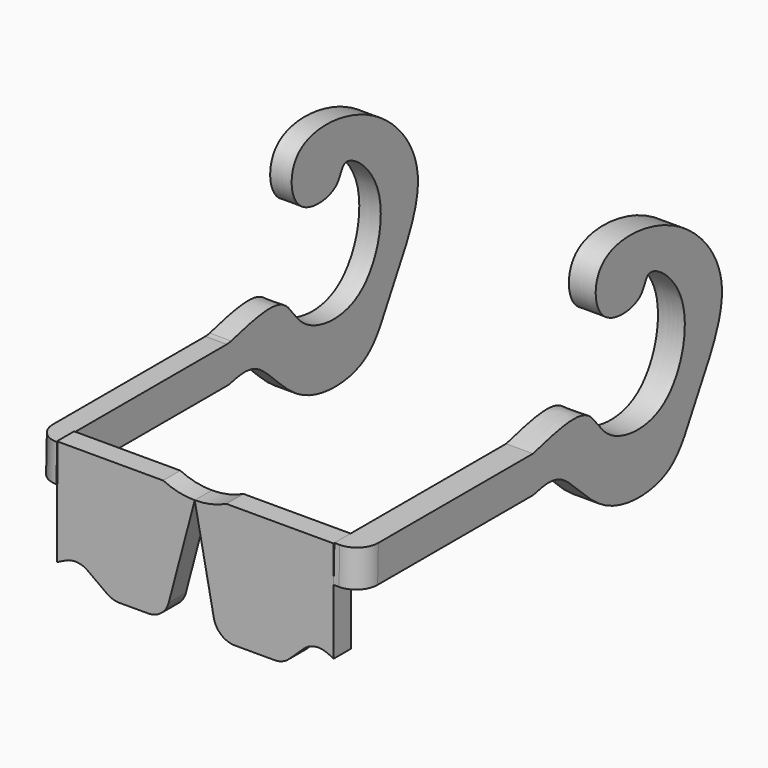
from build123d import *

# Parameters (mm, degrees)
F1_DEPTH  = 5.08
F2_R      = 5.08
F5_DEPTH  = 5.08
F6_R      = 5.08
F7_DEPTH  = 5.08
F8_R      = 5.08
F10_DEPTH = 6.35
F13_R     = 5.07999
F13_2_R   = 5.07999


# Not quite as in the source:
# - a fillet or chamfer is up to 0.001 mm smaller than in the source, because OpenCascade refuses the exact size


with BuildPart() as f1:
    # F0 (on Right) → F1 (new body)
    with BuildSketch(Plane.YZ):
        with BuildLine():
            Line((18.7036339194, 8.6590908468), (-32.0963636041, 8.6590908468))
            Line((-32.0963636041, 8.6590908468), (-32.3272719979, 0))
            Line((-32.3272719979, 0), (18.7036339194, 0))
            add(Edge.make_bspline(
                [(18.7036339194, 0), (21.4167571987, 0.6372428688), (28.063204378, 2.1983223451), (38.2300388432, -13.794123064), (60.394257954, -14.0245683867), (66.1356081474, 0.3511655731), (80.1390378808, 20.7639219103), (62.081530643, 42.703292602), (35.8799194646, 44.0152577696), (37.1192454184, 25.9630287506), (51.7035192179, 26.7390904218), (52.0022911902, 35.2566591152), (67.237499067, 23.591799501), (60.3549528626, -1.2699881146), (39.459302681, 1.5144697653), (35.721169059, 13.1969605328), (24.8370419283, 10.2946159712), (18.7036339194, 8.6590908468)],
                knots=[0, 0, 0, 0, 0.0497967219, 0.1219890317, 0.1968295181, 0.2629995162, 0.3449563898, 0.4313803509, 0.5107878584, 0.5685518225, 0.6256466487, 0.6632894265, 0.7266066585, 0.8065697144, 0.8765027399, 0.9304069977, 1, 1, 1, 1], degree=3))
        make_face()
    extrude(amount=F1_DEPTH)

    # F2
    f2_edges = [f1.edges().sort_by_distance(p)[0] for p in [
        (2.54, 18.703634, 8.659091),
        (2.54, 18.703634, 0),
    ]]
    fillet(f2_edges, radius=F2_R)


with BuildPart() as f1_1:
    # F3: moved
    add(f1.part.moved(Location((-67.945, 0, 0))))


with BuildPart() as f5:
    # F4 (on Front) → F5 (new body)
    with BuildSketch(Plane.XZ):
        with BuildLine():
            Line((-14.9614168331, 0), (-40.0890111923, 0))
            Line((-40.0890111923, 0), (-40.0890111923, -25.1734238118))
            Line((-40.0890111923, -25.1734238118), (-35.2357774973, -22.8123925626))
            Line((-35.2357774973, -22.8123925626), (-26.938032, -28.8461418822))
            Line((-26.938032, -28.8461418822), (-14.6433674064, -28.8461418822))
            Line((-14.6433674064, -28.8461418822), (-7.4807084166, -1.673407664))
            ThreePointArc((-7.4807084166, -1.673407664), (-11.3135041202, -1.2499491441), (-14.9614168331, 0))
        make_face()
    extrude(amount=F5_DEPTH)

    # F6
    f6_edges = [f5.edges().sort_by_distance(p)[0] for p in [
        (-26.938032, -2.54, -28.846142),
        (-35.235777, -2.54, -22.812393),
        (-14.643367, -2.54, -28.846142),
    ]]
    fillet(f6_edges, radius=F6_R)


with BuildPart() as f7:
    # F4 (on Front) → F7 (new body)
    with BuildSketch(Plane.XZ):
        with BuildLine():
            ThreePointArc((0, 0), (-3.6479127129, -1.2499491441), (-7.4807084166, -1.673407664))
            Line((-7.4807084166, -1.673407664), (-2.1583844248, -28.8461418822))
            Line((-2.1583844248, -28.8461418822), (13.412274749, -28.8461418822))
            Line((13.412274749, -28.8461418822), (20.7731388509, -21.8942146748))
            Line((20.7731388509, -21.8942146748), (25.4, -23.9929081872))
            Line((25.4, -23.9929081872), (25.4, 0))
            Line((25.4, 0), (0, 0))
        make_face()
    extrude(amount=F7_DEPTH)

    # F8
    f8_edges = [f7.edges().sort_by_distance(p)[0] for p in [
        (20.773139, -2.54, -21.894215),
        (13.412275, -2.54, -28.846142),
        (-2.158384, -2.54, -28.846142),
    ]]
    fillet(f8_edges, radius=F8_R)


with BuildPart() as f10:
    # F9 (on Right) → F10 (new body)
    with BuildSketch(Plane.YZ):
        with BuildLine():
            Line((122.7466847543, 5.5158741027), (71.9466872309, 5.5158741027))
            Line((71.9466872309, 5.5158741027), (71.715778837, -3.1432167441))
            Line((71.715778837, -3.1432167441), (122.7466847543, -3.1432167441))
            add(Edge.make_bspline(
                [(122.7466847543, -3.1432167441), (125.4598080337, -2.5059738753), (132.1062552129, -0.944894399), (142.2730896781, -16.9373398081), (164.437308789, -17.1677851308), (170.1786589823, -2.792051171), (184.1820887158, 17.6207051662), (166.124581478, 39.5600758579), (139.9229702995, 40.8720410255), (141.1622962533, 22.8198120065), (155.7465700529, 23.5958736777), (156.0453420252, 32.1134423711), (171.2805499019, 20.4485827569), (164.3980036975, -4.4132048587), (143.502353516, -1.6287469788), (139.7642198939, 10.0537437887), (128.8800927632, 7.1513992271), (122.7466847543, 5.5158741027)],
                knots=[0, 0, 0, 0, 0.0497967219, 0.1219890317, 0.1968295181, 0.2629995162, 0.3449563898, 0.4313803509, 0.5107878584, 0.5685518225, 0.6256466487, 0.6632894265, 0.7266066585, 0.8065697144, 0.8765027399, 0.9304069977, 1, 1, 1, 1], degree=3))
        make_face()
    extrude(amount=F10_DEPTH)


with BuildPart() as f10_1:
    # F11: moved
    add(f10.part.moved(Location((25.4, -76.835, -5.461))))

    # F13#2 (radius 5.08 in the source; OpenCascade refuses exactly that, so slightly less here)
    f13_2_edges = [f10_1.edges().sort_by_distance(p)[0] for p in [
        (31.75, -5.003767, -4.274671),
    ]]
    fillet(f13_2_edges, radius=F13_2_R)


with BuildPart() as f1_2:
    # F12: moved
    add(f1_1.part.moved(Location((22.86, 26.9875, -8.8265))))

    # F13 (radius 5.08 in the source; OpenCascade refuses exactly that, so slightly less here)
    f13_edges = [f1_2.edges().sort_by_distance(p)[0] for p in [
        (-45.085, -5.224318, -4.496955),
    ]]
    fillet(f13_edges, radius=F13_R)


solid = Compound([f5.part, f7.part, f10_1.part, f1_2.part])
